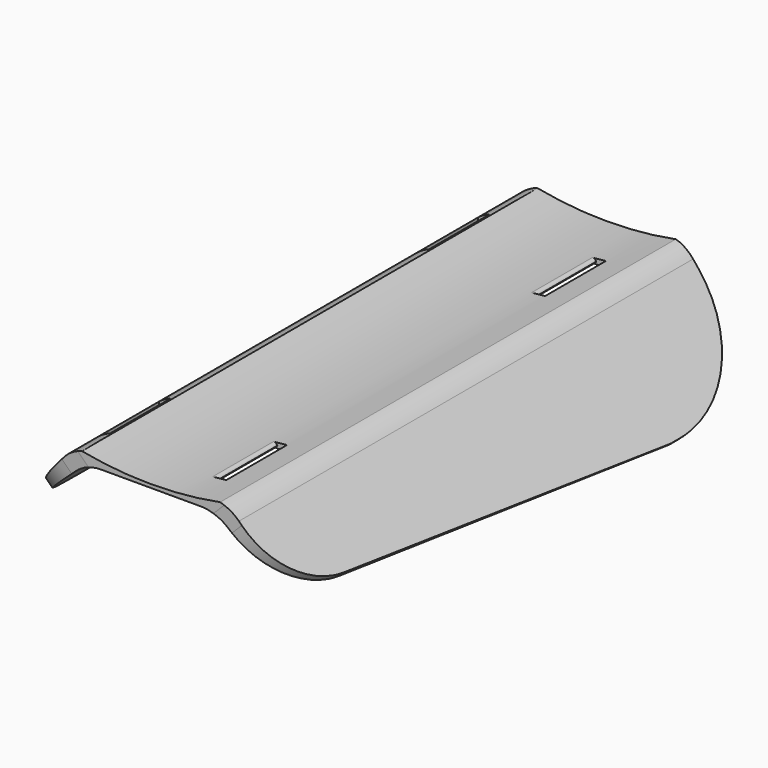
from build123d import *

# Parameters (mm, degrees)
F0_W                   = 40
F0_H                   = 150
F1_DEPTH               = 3
F3_SIZE2               = 2.99999
F3_SIZE                = 2.99999
F4_DEPTH               = 35
DRAFT_F4_DRAFTED_ANGLE = 3
F5_DEPTH               = 35
DRAFT_F5_DRAFTED_ANGLE = 3
F6_R                   = 10
F7_R                   = 30
F8_SIZE2               = 115
F8_SIZE                = 12.5
F8_2_SIZE2             = 115
F8_2_SIZE              = 12.5
F9_R                   = 20
F10_DEPTH              = 150
F11_W                  = 2.5
F11_H                  = 20
F12_DEPTH              = 5
F13_T1_DEPTH           = 20
F13_T3_DEPTH           = 20


# Not quite as in the source:
# - a fillet or chamfer that OpenCascade refuses, or shapes differently, is made with other operations: its cross-section is extruded or revolved along the edge and cut away or added
# - a fillet or chamfer is up to 0.001 mm smaller than in the source, because OpenCascade refuses the exact size
# - an extrude with a draft is written as a straight extrude whose walls are then drafted


with BuildPart() as f1:
    # F0 (on Top) → F1 (new body)
    with BuildSketch(Plane.XY):
        with Locations((20, 75)):
            Rectangle(F0_W, F0_H)
    extrude(amount=F1_DEPTH)

    # F3 (size 3 and 3 in the source; OpenCascade refuses exactly that, so slightly less here)
    f3_edges = [f1.edges().sort_by_distance(p)[0] for p in [
        (0, 75, 0),
        (40, 75, 0),
    ]]
    chamfer(f3_edges, length=F3_SIZE, length2=F3_SIZE2)


with BuildPart() as f4_drafted:
    # F4 (new): a face of the model
    f4_faces = [f1.part.faces().sort_by_distance(p)[0] for p in [
        (38.500005, 75, 1.499995),
    ]]
    extrude(f4_faces, amount=F4_DEPTH)

    # draft_F4_drafted
    draft_f4_drafted_walls = [f4_drafted.faces().sort_by_distance(p)[0] for p in [
        (54.9991632277, 0, -14.9991632277),
        (56.4991582277, 75, -13.4991682277),
        (53.4991682277, 75, -16.4991582277),
        (54.9991632277, 150, -14.9991632277),
    ]]
    draft(draft_f4_drafted_walls, neutral_plane=Plane(origin=(38.500005, 75, 1.499995), x_dir=(0, 1, 0), z_dir=(0.7071067812, 0, -0.7071067812)), angle=DRAFT_F4_DRAFTED_ANGLE)


with BuildPart() as f1_1:
    add(f1.part)

    # join_F4_drafted: union F4_drafted
    add(f4_drafted.part)


with BuildPart() as f5_drafted:
    # F5 (new): a face of the model
    f5_faces = [f1_1.part.faces().sort_by_distance(p)[0] for p in [
        (1.499995, 75, 1.499995),
    ]]
    extrude(f5_faces, amount=F5_DEPTH)

    # draft_F5_drafted
    draft_f5_drafted_walls = [f5_drafted.faces().sort_by_distance(p)[0] for p in [
        (-14.9991632277, 150, -14.9991632277),
        (-16.4991582277, 75, -13.4991682277),
        (-13.4991682277, 75, -16.4991582277),
        (-14.9991632277, 0, -14.9991632277),
    ]]
    draft(draft_f5_drafted_walls, neutral_plane=Plane(origin=(1.499995, 75, 1.499995), x_dir=(0, -1, 0), z_dir=(-0.7071067812, 0, -0.7071067812)), angle=DRAFT_F5_DRAFTED_ANGLE)


with BuildPart() as f1_2:
    add(f1_1.part)

    # join_F5_drafted: union F5_drafted
    add(f5_drafted.part)

    # F6 (call 1 of 4: OpenCascade refuses the feature's edges together)
    f6_edges = [f1_2.edges().sort_by_distance(p)[0] for p in [
        (40, 75, 2.99999),
    ]]
    fillet(f6_edges, radius=F6_R)

    # F6#2 (call 2 of 4)
    f6_2_edges = [f1_2.edges().sort_by_distance(p)[0] for p in [
        (0, 75, 3),
    ]]
    fillet(f6_2_edges, radius=F6_R)

    # F6#3 (call 3 of 4)
    f6_3_edges = [f1_2.edges().sort_by_distance(p)[0] for p in [
        (37.00001, 75, 0),
    ]]
    fillet(f6_3_edges, radius=F6_R)

    # F6#4 (call 4 of 4)
    f6_4_edges = [f1_2.edges().sort_by_distance(p)[0] for p in [
        (2.99999, 75, 0),
    ]]
    fillet(f6_4_edges, radius=F6_R)

    # F7
    f7_edges = [f1_2.edges().sort_by_distance(p)[0] for p in [
        (-23.248742, 148.165728, -23.248742),
        (63.248742, 148.165728, -23.248742),
    ]]
    fillet(f7_edges, radius=F7_R)

    # F8
    f8_edges = [f1_2.edges().sort_by_distance(p)[0] for p in [
        (-23.248742, 1.834272, -23.248742),
    ]]
    f8_side = f1_2.faces().sort_by_distance((-7.741742, 0.688012, -7.824141))[0]
    chamfer(f8_edges, length=F8_SIZE, length2=F8_SIZE2, reference=f8_side)

    # F8#2
    f8_2_edges = [f1_2.edges().sort_by_distance(p)[0] for p in [
        (63.248742, 1.834272, -23.248742),
    ]]
    f8_2_side = f1_2.faces().sort_by_distance((47.741742, 0.688012, -7.824141))[0]
    chamfer(f8_2_edges, length=F8_2_SIZE, length2=F8_2_SIZE2, reference=f8_2_side)

    # F9
    f9_edges = [f1_2.edges().sort_by_distance(p)[0] for p in [
        (54.422021, 1.180073, -14.422021),
        (-14.422021, 1.180073, -14.422021),
    ]]
    fillet(f9_edges, radius=F9_R)

    # F2 (on face) → F10 (cut, through all)
    with BuildSketch(Plane(origin=(0, 150, 0), x_dir=(-1, 0, 0), z_dir=(0, 1, 0))):
        with BuildLine():
            Line((0, 3), (-40, 3))
            ThreePointArc((-40, 3), (-20, 0.8950469189), (0, 3))
        make_face()
    extrude(amount=-F10_DEPTH, mode=Mode.SUBTRACT)

    # F11 (on Top) → F12 (cut, symmetric)
    with BuildSketch(Plane.XY):
        with Locations((-0.5994591439, 125)):
            Rectangle(F11_W, F11_H)
        with Locations((30.5859880339, 125)):
            Rectangle(F11_W, F11_H)
        with Locations((30.5859880339, 19.999745685)):
            Rectangle(F11_W, F11_H)
        with Locations((-0.5994591439, 19.999745685)):
            Rectangle(F11_W, F11_H)
    extrude(amount=F12_DEPTH, both=True, mode=Mode.SUBTRACT)

    # F13: fillet of radius 1 on 8 edges, made by hand

    # F13_s2 → F13_t1 (cut)
    with BuildSketch(Plane.XZ.offset(-135)):
        with BuildLine():
            ThreePointArc((2.1221853555, -1.182112123), (1.136558609, -1.1581241571), (0.6505408561, -0.3003233353))
            Line((0.6505408561, -0.3003233353), (0.6505408561, -2.1445847716))
            ThreePointArc((0.6505408561, -2.1445847716), (1.3651665014, -1.6309383146), (2.1221853555, -1.182112123))
        make_face()
        with BuildLine():
            ThreePointArc((28.3359880339, 0), (29.0430948151, 0.2928932188), (29.3359880339, 1))
            Line((29.3359880339, 1), (29.3359880339, 0))
            Line((29.3359880339, 0), (28.3359880339, 0))
        make_face()
        with BuildLine():
            ThreePointArc((28.250108863, 1.2499587737), (29.0120504678, 0.9904975569), (29.3359880339, 0.2536532141))
            Line((29.3359880339, 0.2536532141), (29.3359880339, 1.3497708495))
            ThreePointArc((29.3359880339, 1.3497708495), (28.7931900713, 1.2983240635), (28.250108863, 1.2499587737))
        make_face()
        with BuildLine():
            ThreePointArc((1.3392347448, 2.5030968905), (0.8408167946, 2.1395980265), (0.6505408561, 1.5527872015))
            Line((0.6505408561, 1.5527872015), (0.6505408561, 2.2491436853))
            ThreePointArc((0.6505408561, 2.2491436853), (0.9925569178, 2.3824413919), (1.3392347448, 2.5030968905))
        make_face()
    extrude(amount=F13_T1_DEPTH, mode=Mode.SUBTRACT)

    # F13_s4 → F13_t3 (cut)
    with BuildSketch(Plane.XZ.offset(-29.999745685)):
        with BuildLine():
            ThreePointArc((2.1221853555, -1.182112123), (1.136558609, -1.1581241571), (0.6505408561, -0.3003233353))
            Line((0.6505408561, -0.3003233353), (0.6505408561, -2.1445847716))
            ThreePointArc((0.6505408561, -2.1445847716), (1.3651665014, -1.6309383146), (2.1221853555, -1.182112123))
        make_face()
        with BuildLine():
            ThreePointArc((28.3359880339, 0), (29.0430948151, 0.2928932188), (29.3359880339, 1))
            Line((29.3359880339, 1), (29.3359880339, 0))
            Line((29.3359880339, 0), (28.3359880339, 0))
        make_face()
        with BuildLine():
            ThreePointArc((28.250108863, 1.2499587737), (29.0120504678, 0.9904975569), (29.3359880339, 0.2536532141))
            Line((29.3359880339, 0.2536532141), (29.3359880339, 1.3497708495))
            ThreePointArc((29.3359880339, 1.3497708495), (28.7931900713, 1.2983240635), (28.250108863, 1.2499587737))
        make_face()
        with BuildLine():
            ThreePointArc((1.3392347448, 2.5030968905), (0.8408167946, 2.1395980265), (0.6505408561, 1.5527872015))
            Line((0.6505408561, 1.5527872015), (0.6505408561, 2.2491436853))
            ThreePointArc((0.6505408561, 2.2491436853), (0.9925569178, 2.3824413919), (1.3392347448, 2.5030968905))
        make_face()
    extrude(amount=F13_T3_DEPTH, mode=Mode.SUBTRACT)


solid = f1_2.part
